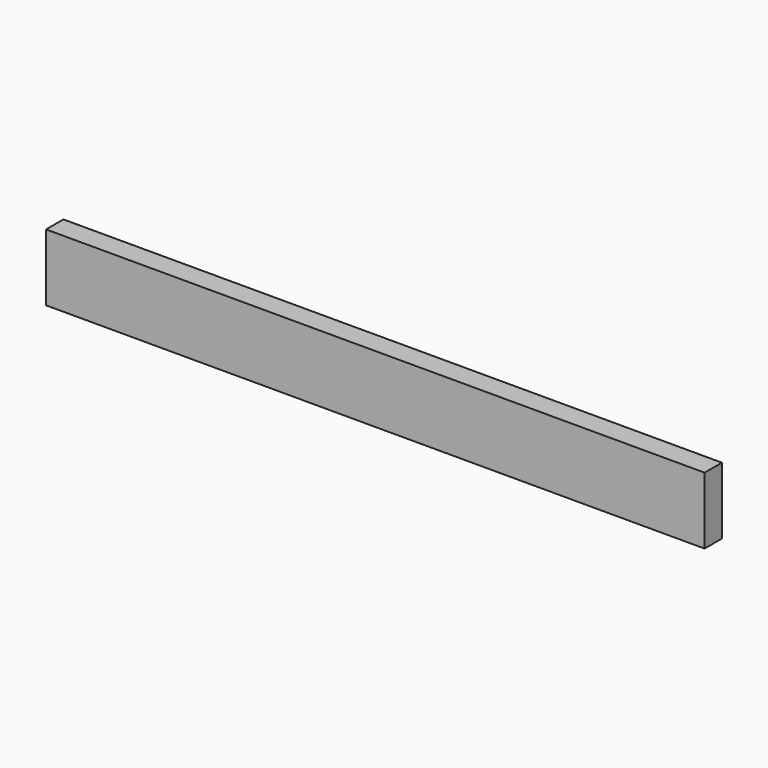
from build123d import *

# Parameters (mm, degrees)
F0_W     = 75.6163597107
F0_H     = 15.3191536665
F0_W_2   = 75.2519443631
F1_DEPTH = 4.9654152244


# Not quite as in the source:
# - the program builds the solid bodies; features that only make, move or delete a surface that nothing else refers to are left out


with BuildPart() as f1:
    # F0 (on Front) → F1 (new body)
    with BuildSketch(Plane.XZ):
        with Locations((37.8081798553, -7.6595768332)):
            Rectangle(F0_W, F0_H)
        with Locations((-37.6259721816, -7.6595768332)):
            Rectangle(F0_W_2, F0_H)
    extrude(amount=F1_DEPTH)


solid = f1.part
